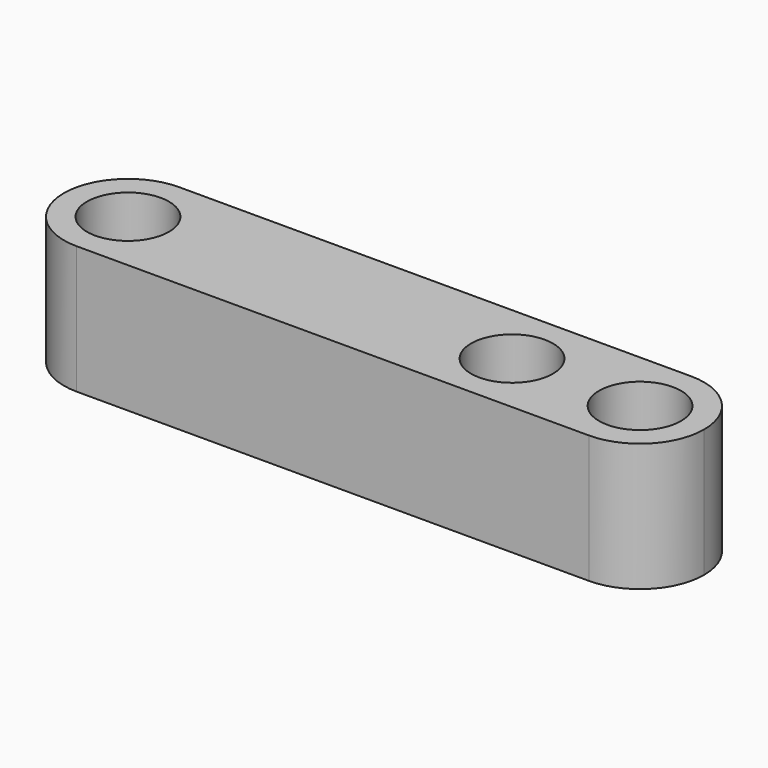
from build123d import *

# Parameters (mm, degrees)
F0_W     = 39.6875
F0_H     = 7.9375
F0_R     = 2.54
F1_DEPTH = 7.9375
F2_R     = 3.96874


# Not quite as in the source:
# - a fillet or chamfer is up to 0.001 mm smaller than in the source, because OpenCascade refuses the exact size


with BuildPart() as f1:
    # F0 (on Top) → F1 (new body)
    with BuildSketch(Plane.XY):
        with Locations((19.84375, -3.96875)):
            Rectangle(F0_W, F0_H)
        with Locations((3.96875, -3.96875)):
            Circle(F0_R, mode=Mode.SUBTRACT)
        with Locations((27.78125, -3.96875)):
            Circle(F0_R, mode=Mode.SUBTRACT)
        with Locations((35.71875, -3.96875)):
            Circle(F0_R, mode=Mode.SUBTRACT)
    extrude(amount=F1_DEPTH)

    # F2 (radius 3.96875 in the source; OpenCascade refuses exactly that, so slightly less here)
    f2_edges = [f1.edges().sort_by_distance(p)[0] for p in [
        (0, 0, 3.96875),
        (0, -7.9375, 3.96875),
        (39.6875, -7.9375, 3.96875),
        (39.6875, 0, 3.96875),
    ]]
    fillet(f2_edges, radius=F2_R)


solid = f1.part
